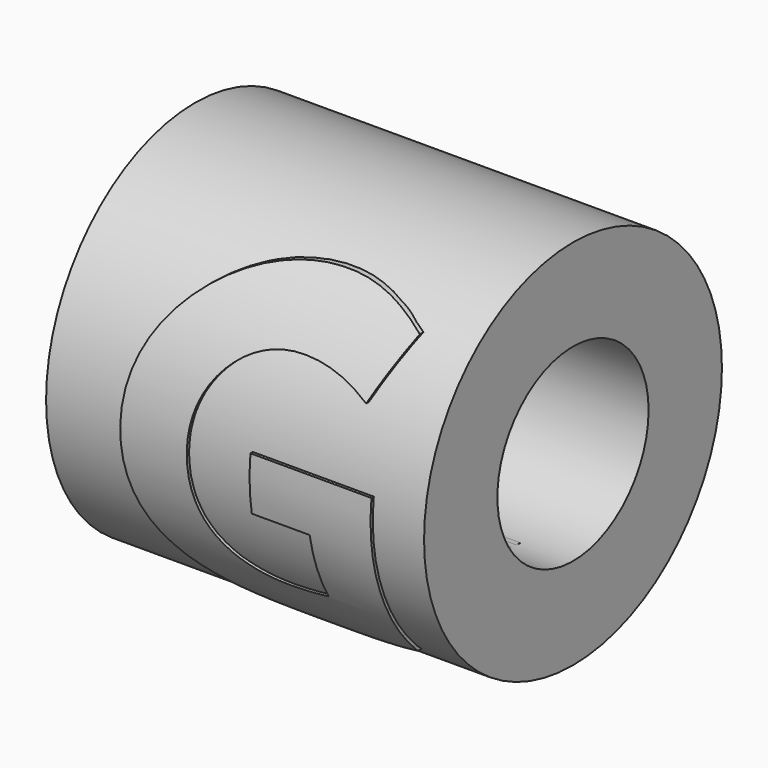
from build123d import *

# Parameters (mm, degrees)
F0_R         = 1
F0_R_2       = 0.985
F0_R_3       = 0.5
F1_DEPTH     = 2
F2_TEXT_SIZE = 2.2604994431
F3_REACH     = 3.1238742156
F4_DEPTH     = 2


# Not quite as in the source:
# - Text() gives the source's letters only with a copy of the font that has no kerning and outlines rounded to 1/6400 em; it was checked with that copy


with BuildPart() as f1:
    # F0 (on Right) → F1 (new body)
    with BuildSketch(Plane.YZ):
        Circle(F0_R)
        Circle(F0_R_2, mode=Mode.SUBTRACT)
        Circle(F0_R_2)
        Circle(F0_R_3, mode=Mode.SUBTRACT)
    extrude(amount=F1_DEPTH)

    f3_end = f1.faces().sort_by_distance((1, -1, 0))[0]
    # F2 (on Front) → F3 (intersect, up to a face of the model that its end follows)
    with BuildSketch(Plane.XZ):
        with Locations((0.2728080435, -0.7963191019)):
            Text('G', F2_TEXT_SIZE, font='Open Sans', font_style=FontStyle.BOLD, text_align=(TextAlign.LEFT, TextAlign.BOTTOM))
    f3_long = extrude(amount=F3_REACH, mode=Mode.PRIVATE)
    add(split(f3_long, bisect_by=f3_end, keep=Keep.BOTTOM, mode=Mode.PRIVATE), mode=Mode.INTERSECT)


with BuildPart() as f4:
    # F0 (on Right) → F4 (new body)
    with BuildSketch(Plane.YZ):
        Circle(F0_R_2)
        Circle(F0_R_3, mode=Mode.SUBTRACT)
    extrude(amount=F4_DEPTH)


solid = Compound([f1.part, f4.part])
